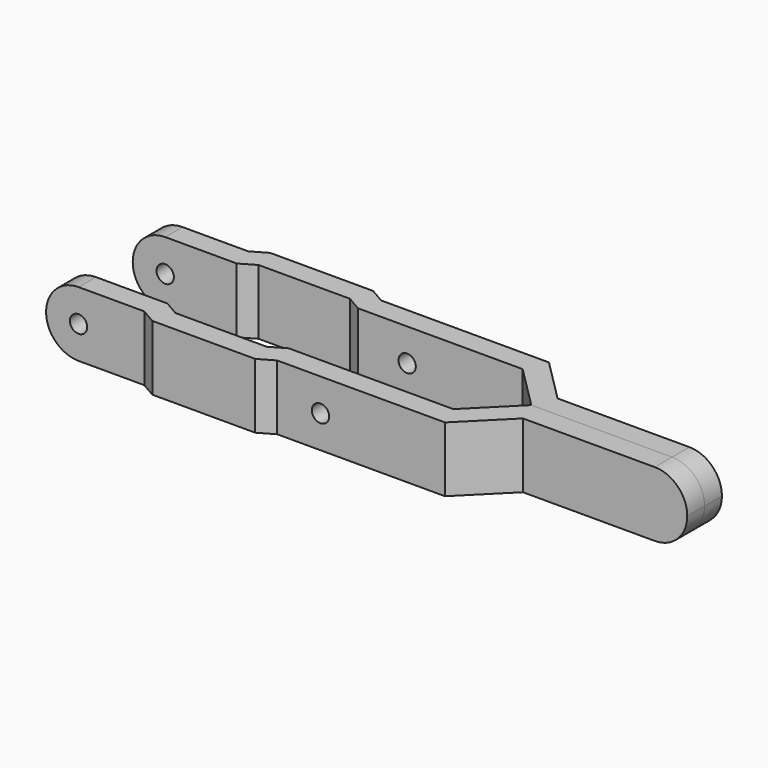
from build123d import *

# Parameters (mm, degrees)
F1_DEPTH = 19.05
F2_R     = 9.52499
F3_R     = 2.54
F4_DEPTH = 25.4


# Not quite as in the source:
# - a fillet or chamfer is up to 0.001 mm smaller than in the source, because OpenCascade refuses the exact size


with BuildPart() as f1:
    # F0 (on Top) → F1 (new body)
    with BuildSketch(Plane.XY):
        Polygon((27.94, -12.7), (-2.54, -12.7), (-2.54, -19.05), (26.2385226281, -19.05), (30.6379316793, -21.59), (60.8020683207, -21.59), (65.2014773719, -19.05), (114.3902561211, -19.05), (127.0902561211, -6.35), (175.26, -6.35), (175.26, 0), (124.46, 0), (111.76, -12.7), (63.5, -12.7), (59.1005909488, -15.24), (32.3394090512, -15.24), align=None)
    extrude(amount=F1_DEPTH)

    # F2 (radius 9.525 in the source; OpenCascade refuses exactly that, so slightly less here)
    f2_edges = [f1.edges().sort_by_distance(p)[0] for p in [
        (-2.54, -15.875, 19.05),
        (-2.54, -15.875, 0),
        (175.26, -3.175, 19.05),
        (175.26, -3.175, 0),
    ]]
    fillet(f2_edges, radius=F2_R)

    # F3 (on Front) → F4 (cut)
    with BuildSketch(Plane.XZ):
        with Locations((6.985, 9.525)):
            Circle(F3_R)
        with Locations((77.9014773719, 9.525)):
            Circle(F3_R)
    extrude(amount=F4_DEPTH, mode=Mode.SUBTRACT)


with BuildPart() as f5_1:
    # F5: instance of F1
    add(f1.part.mirror(Plane.XZ))


solid = Compound([f1.part, f5_1.part])
